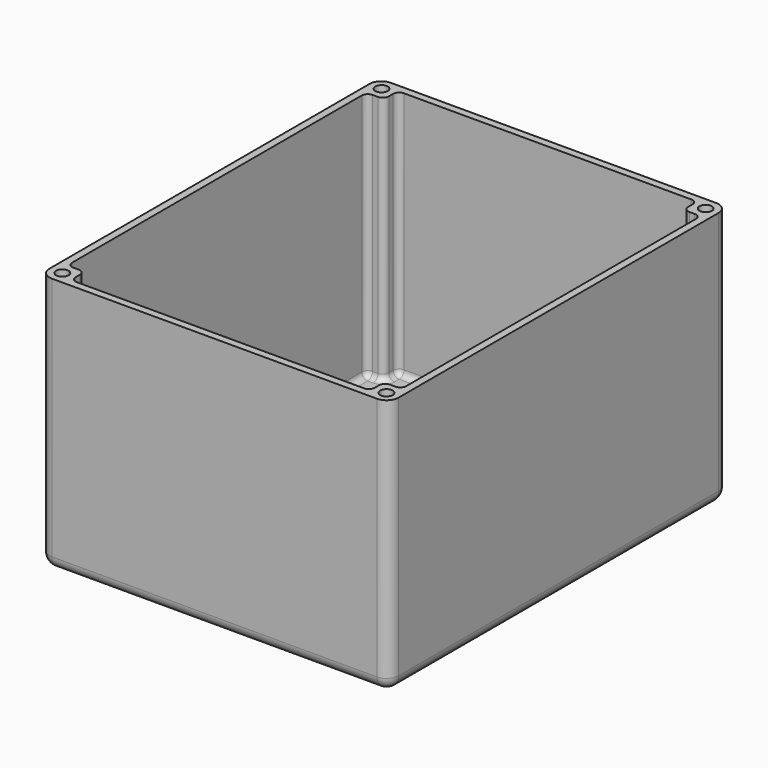
from build123d import *

# Parameters (mm, degrees)
F0_W     = 70
F0_H     = 85
F0_R     = 1.5
F0_W_2   = 24.796
F0_H_2   = 8.8934727723
F0_R_2   = 19
F1_DEPTH = 1.5
F2_W     = 70
F2_H     = 85
F3_DEPTH = 50
F4_R     = 1.25
F5_DEPTH = 15
F6_R     = 2.5
F7_DEPTH = 3
F8_R     = 0.75
F9_DEPTH = 2.4
F10_R    = 2.4
F11_F1_R = 1.2
F11_F2_R = 1.2


with BuildPart() as f1:
    # F0 (on Top) → F1 (new body)
    with BuildSketch(Plane.XY):
        with Locations((0, -7.5)):
            Rectangle(F0_W, F0_H)
        with Locations((-16.6170093579, -16.6170093579)):
            Circle(F0_R, mode=Mode.SUBTRACT)
        with Locations((0, -33.3067363862)):
            Rectangle(F0_W_2, F0_H_2, mode=Mode.SUBTRACT)
        with Locations((16.6170093579, -16.6170093579)):
            Circle(F0_R, mode=Mode.SUBTRACT)
        with Locations((-16.6170093579, 16.6170093579)):
            Circle(F0_R, mode=Mode.SUBTRACT)
        Circle(F0_R_2, mode=Mode.SUBTRACT)
        with Locations((16.6170093579, 16.6170093579)):
            Circle(F0_R, mode=Mode.SUBTRACT)
    extrude(amount=F1_DEPTH)

    # F2 (on face) → F3 (join)
    with BuildSketch(Plane.XY.offset(1.5)):
        with Locations((0, -7.5)):
            Rectangle(F2_W, F2_H)
        Polygon((-30, 30), (-30, 33.5), (30, 33.5), (30, 30), (33.5, 30), (33.5, -45), (30, -45), (30, -48.5), (-30, -48.5), (-30, -45), (-33.5, -45), (-33.5, 30), align=None, mode=Mode.SUBTRACT)
    extrude(amount=F3_DEPTH)

    # F4 (on face) → F5 (cut)
    with BuildSketch(Plane.XY.offset(51.5)):
        with Locations((-32.5, 32.5)):
            Circle(F4_R)
        with Locations((32.5, -47.5)):
            Circle(F4_R)
        with Locations((32.5, 32.5)):
            Circle(F4_R)
        with Locations((-32.5, -47.5)):
            Circle(F4_R)
    extrude(amount=-F5_DEPTH, mode=Mode.SUBTRACT)

    # F6 (on face) → F7 (join)
    with BuildSketch(Plane.XY):
        with Locations((-16.5714677423, -23.966986686)):
            Circle(F6_R)
        with Locations((12.4001037329, -23.9952448756)):
            Circle(F6_R)
        with Locations((12.3935937881, -44.0698005259)):
            Circle(F6_R)
        with Locations((-16.5627133101, -44.0643951297)):
            Circle(F6_R)
    extrude(amount=F7_DEPTH)

    # F8 (on face) → F9 (cut)
    with BuildSketch(Plane.XY.offset(3)):
        with Locations((-16.5714677423, -23.966986686)):
            Circle(F8_R)
        with Locations((12.4562103301, -23.9926725626)):
            Circle(F8_R)
        with Locations((12.4562103301, -44.1322289407)):
            Circle(F8_R)
        with Locations((-16.5714677423, -44.1322289407)):
            Circle(F8_R)
    extrude(amount=-F9_DEPTH, mode=Mode.SUBTRACT)

    # F10
    f10_edges = [f1.edges().sort_by_distance(p)[0] for p in [
        (-35, 35, 25.75),
        (-35, -50, 25.75),
        (-35, -7.5, 0),
        (0, 35, 0),
        (35, -7.5, 0),
        (0, -50, 0),
        (35, 35, 25.75),
        (35, -50, 25.75),
    ]]
    fillet(f10_edges, radius=F10_R)

    # F11: fillet of radius 1.2 on 23 edges, made by hand

    # F11_f1
    f11_f1_edges = [f1.edges().sort_by_distance(p)[0] for p in [
        (-30, 30, 26.5),
        (30, 30, 26.5),
        (-30, -45, 26.5),
        (30, -45, 26.5),
    ]]
    fillet(f11_f1_edges, radius=F11_F1_R)

    # F11_f2
    f11_f2_edges = [f1.edges().sort_by_distance(p)[0] for p in [
        (0, 33.5, 1.5),
        (-30, 32.35, 1.5),
        (-32.35, 30, 1.5),
        (-30, 33.5, 26.5),
        (-33.5, 30, 26.5),
        (-33.5, -7.5, 1.5),
        (30, 32.35, 1.5),
        (32.35, 30, 1.5),
        (30, 33.5, 26.5),
        (33.5, 30, 26.5),
        (33.5, -7.5, 1.5),
        (-33.5, -45, 26.5),
        (-32.35, -45, 1.5),
        (-30, -48.5, 26.5),
        (0, -48.5, 1.5),
        (30, -47.35, 1.5),
        (32.35, -45, 1.5),
        (33.5, -45, 26.5),
        (30, -48.5, 26.5),
        (30.3514718626, -45.3514718626, 1.5),
        (-30.3514718626, -45.3514718626, 1.5),
        (30.3514718626, 30.3514718626, 1.5),
        (-30.3514718626, 30.3514718626, 1.5),
    ]]
    fillet(f11_f2_edges, radius=F11_F2_R)


solid = f1.part
